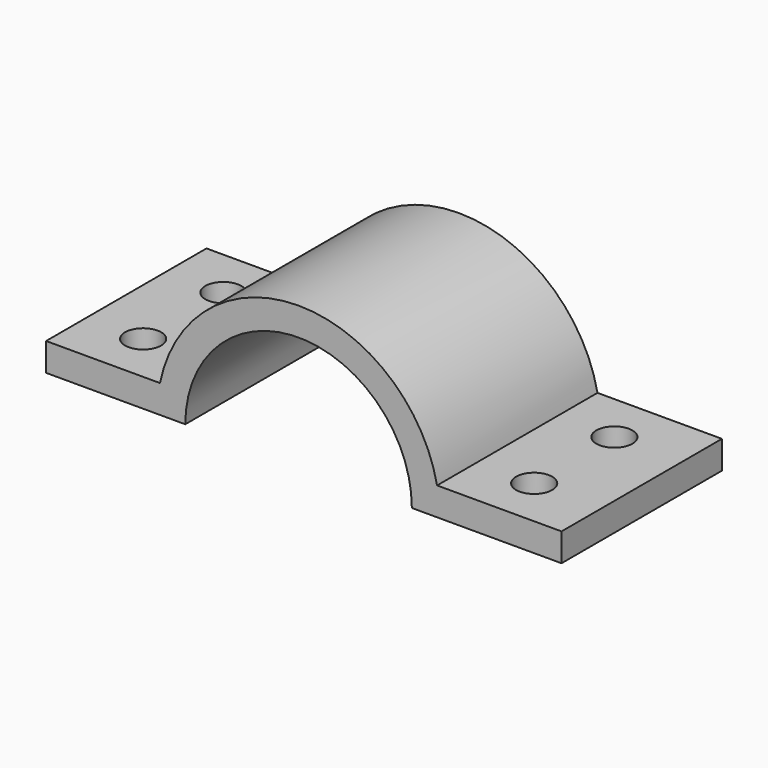
from build123d import *

# Parameters (mm, degrees)
F1_DEPTH = 25
F2_R     = 4.5
F3_DEPTH = 7.001


# Not quite as in the source:
# - a pattern or mirror of a feature is missing from the dataset's text; its kind, count and spacing are read off the source's solid


with BuildPart() as f1:
    # F0 (on Front) → F1 (new body, symmetric)
    with BuildSketch(Plane.XZ):
        with BuildLine():
            ThreePointArc((-28.2506073348, 0), (0, 28.2506073348), (28.2506073348, 0))
            Line((28.2506073348, 0), (65.5786693096, 0))
            Line((65.5786693096, 0), (65.5786693096, 7))
            Line((65.5786693096, 7), (34.5485935672, 7))
            ThreePointArc((34.5485935672, 7), (0, 35.2506073348), (-34.5485935672, 7))
            Line((-34.5485935672, 7), (-62.9629269242, 7))
            Line((-62.9629269242, 7), (-62.9629269242, 0))
            Line((-62.9629269242, 0), (-28.2506073348, 0))
        make_face()
    extrude(amount=F1_DEPTH, both=True)

    # F2 (on face) → F3 (cut, through all)
    with BuildSketch(Plane.XY.offset(7)):
        with Locations((-48.7557602457, -12.5)):
            Circle(F2_R)
        with Locations((-48.7557602457, 12.5)):
            Circle(F2_R)
    f3 = extrude(amount=-F3_DEPTH, mode=Mode.SUBTRACT)

    # F3_copies: F3 across plane
    add(f3.mirror(Plane(origin=(0, 0, 0), x_dir=(0, 0, 1), z_dir=(1, 0, 0))), mode=Mode.SUBTRACT)


solid = f1.part
